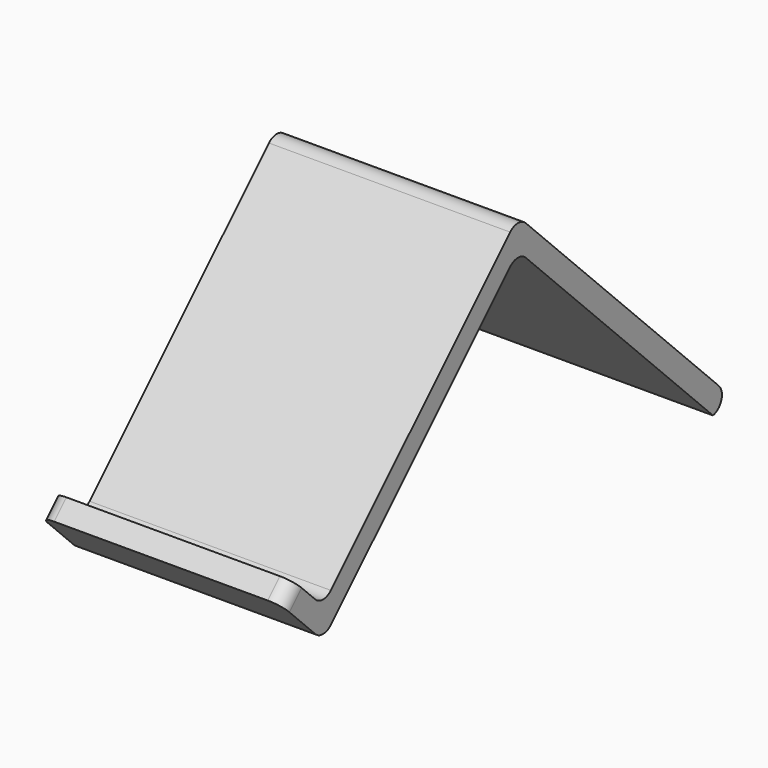
from build123d import *

# Parameters (mm, degrees)
F1_DEPTH     = 88.9
F2_T1_DEPTH  = 88.9
F2_T3_DEPTH  = 88.9
F2_T5_DEPTH  = 149.5881510316
F2_T7_DEPTH  = 114.3
F2_T9_DEPTH  = 33.3375
F2_T11_DEPTH = 33.3375
F2_T13_DEPTH = 114.3


# Not quite as in the source:
# - a fillet or chamfer that OpenCascade refuses, or shapes differently, is made with other operations: its cross-section is extruded or revolved along the edge and cut away or added


with BuildPart() as f1:
    # F0 (on Right) → F1 (new body)
    with BuildSketch(Plane.YZ):
        Polygon((-11.2253201513, 0), (0, 0), (-101.027881362, 101.027881362), (-190.8304425727, 11.2253201513), (-204.3008267543, 24.6957043329), (-209.91348683, 19.0830442573), (-190.8304425727, 0), (-101.027881362, 89.8025612107), align=None)
    extrude(amount=-F1_DEPTH)

    # F2: fillet of radius 5.08 on 7 edges, made by hand

    # F2_s2 → F2_t1 (join)
    with BuildSketch(Plane.YZ.offset(-88.9)):
        with BuildLine():
            ThreePointArc((-97.4357789136, 86.2104587623), (-101.027881362, 87.6983563138), (-104.6199838105, 86.2104587623))
            Line((-104.6199838105, 86.2104587623), (-101.027881362, 89.8025612107))
            Line((-101.027881362, 89.8025612107), (-97.4357789136, 86.2104587623))
        make_face()
    extrude(amount=F2_T1_DEPTH)

    # F2_s4 → F2_t3 (join)
    with BuildSketch(Plane.YZ.offset(-88.9)):
        with BuildLine():
            ThreePointArc((-187.2383401243, 14.8174225998), (-190.8304425727, 13.3295250482), (-194.4225450211, 14.8174225998))
            Line((-194.4225450211, 14.8174225998), (-190.8304425727, 11.2253201513))
            Line((-190.8304425727, 11.2253201513), (-187.2383401243, 14.8174225998))
        make_face()
    extrude(amount=F2_T3_DEPTH)

    # F2_s6 → F2_t5 (cut)
    with BuildSketch(Plane.YZ.offset(-119.2440755158)):
        with BuildLine():
            ThreePointArc((-11.2253201513, 0), (-7.3196509923, 3.4955502605), (-8.5826006264, 8.5826006264))
            Line((-8.5826006264, 8.5826006264), (0, 0))
            Line((0, 0), (-11.2253201513, 0))
        make_face()
    extrude(amount=F2_T5_DEPTH, mode=Mode.SUBTRACT)

    # F2_s8 → F2_t7 (cut)
    with BuildSketch(Plane.YZ.offset(-101.6)):
        with BuildLine():
            ThreePointArc((-104.6199838105, 97.4357789136), (-101.027881362, 98.9236764652), (-97.4357789136, 97.4357789136))
            Line((-97.4357789136, 97.4357789136), (-101.027881362, 101.027881362))
            Line((-101.027881362, 101.027881362), (-104.6199838105, 97.4357789136))
        make_face()
    extrude(amount=F2_T7_DEPTH, mode=Mode.SUBTRACT)

    # F2_s10 → F2_t9 (cut)
    with BuildSketch(Plane(origin=(0, -80.8223050896, -80.8223050896), x_dir=(1, 0, 0), z_dir=(0, -0.7071067812, -0.7071067812))):
        with BuildLine():
            ThreePointArc((0, 156.845), (-1.4878975516, 160.4371024484), (-5.08, 161.925))
            Line((-5.08, 161.925), (0, 161.925))
            Line((0, 161.925), (0, 156.845))
        make_face()
    extrude(amount=F2_T9_DEPTH, mode=Mode.SUBTRACT)

    # F2_s12 → F2_t11 (cut)
    with BuildSketch(Plane(origin=(0, -80.8223050896, -80.8223050896), x_dir=(1, 0, 0), z_dir=(0, -0.7071067812, -0.7071067812))):
        with BuildLine():
            ThreePointArc((-88.9, 156.845), (-87.4121024484, 160.4371024484), (-83.82, 161.925))
            Line((-83.82, 161.925), (-88.9, 161.925))
            Line((-88.9, 161.925), (-88.9, 156.845))
        make_face()
    extrude(amount=F2_T11_DEPTH, mode=Mode.SUBTRACT)

    # F2_s14 → F2_t13 (cut)
    with BuildSketch(Plane.YZ.offset(-101.6)):
        with BuildLine():
            ThreePointArc((-187.2383401243, 3.5921024484), (-190.8304425727, 2.1042048969), (-194.4225450211, 3.5921024484))
            Line((-194.4225450211, 3.5921024484), (-190.8304425727, 0))
            Line((-190.8304425727, 0), (-187.2383401243, 3.5921024484))
        make_face()
    extrude(amount=F2_T13_DEPTH, mode=Mode.SUBTRACT)


solid = f1.part
